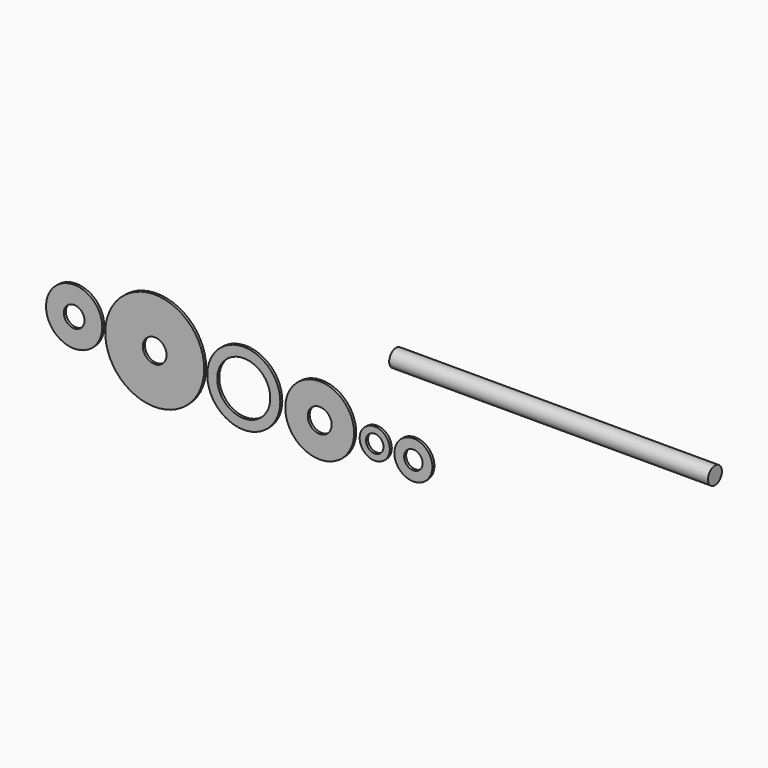
from build123d import *

# Parameters (mm, degrees)
F0_R     = 18.1687180168
F0_R_2   = 8.8190592327
F1_DEPTH = 2.38125
F0_R_3   = 14.4040085197
F0_R_4   = 8.3616203188
F0_R_5   = 32.910330078
F0_R_6   = 11.4321100003
F0_R_7   = 34.9237905831
F0_R_8   = 25.330278317
F0_R_9   = 47.2792187039
F0_R_10  = 11.3237611098
F0_R_11  = 26.8812365552
F0_R_12  = 9.8757429668
F2_R     = 8.3083314945
F3_DEPTH = 304.8


# Not quite as in the source:
# - a length typed as a fraction of an inch, garbled in the dataset ("3 / 203.2 mm" for 3/8 in), is restored


with BuildPart() as f1:
    # F0 (on Front) → F1 (new body)
    with BuildSketch(Plane.XZ):
        with Locations((174.3635833263, 50.7673621178)):
            Circle(F0_R)
        with Locations((174.3635833263, 50.7673621178)):
            Circle(F0_R_2, mode=Mode.SUBTRACT)
    extrude(amount=F1_DEPTH)


with BuildPart() as f1b:
    # F0 (on Front) → F1, piece 2 (new body)
    with BuildSketch(Plane.XZ):
        with Locations((137.4451422389, 52.4887427962)):
            Circle(F0_R_3)
        with Locations((137.4451422389, 52.4887427962)):
            Circle(F0_R_4, mode=Mode.SUBTRACT)
    extrude(amount=F1_DEPTH)


with BuildPart() as f1c:
    # F0 (on Front) → F1, piece 3 (new body)
    with BuildSketch(Plane.XZ):
        with Locations((84.8133870552, 54.9427815848)):
            Circle(F0_R_5)
        with Locations((84.8133870552, 54.9427815848)):
            Circle(F0_R_6, mode=Mode.SUBTRACT)
    extrude(amount=F1_DEPTH)


with BuildPart() as f1d:
    # F0 (on Front) → F1, piece 4 (new body)
    with BuildSketch(Plane.XZ):
        with Locations((12.2279077768, 58.3271943033)):
            Circle(F0_R_7)
        with Locations((12.2279077768, 58.3271943033)):
            Circle(F0_R_8, mode=Mode.SUBTRACT)
    extrude(amount=F1_DEPTH)


with BuildPart() as f1e:
    # F0 (on Front) → F1, piece 5 (new body)
    with BuildSketch(Plane.XZ):
        with Locations((-72.893794205, 62.2961282233)):
            Circle(F0_R_9)
        with Locations((-72.893794205, 62.2961282233)):
            Circle(F0_R_10, mode=Mode.SUBTRACT)
    extrude(amount=F1_DEPTH)


with BuildPart() as f1f:
    # F0 (on Front) → F1, piece 6 (new body)
    with BuildSketch(Plane.XZ):
        with Locations((-149.9077677727, 65.8870264888)):
            Circle(F0_R_11)
        with Locations((-149.9077677727, 65.8870264888)):
            Circle(F0_R_12, mode=Mode.SUBTRACT)
    extrude(amount=F1_DEPTH)


with BuildPart() as f3:
    # F2 (on Right) → F3 (new body)
    with BuildSketch(Plane.YZ):
        with Locations((194.9509978294, 0)):
            Circle(F2_R)
    extrude(amount=F3_DEPTH)


solid = Compound([f1.part, f1b.part, f1c.part, f1d.part, f1e.part, f1f.part, f3.part])
